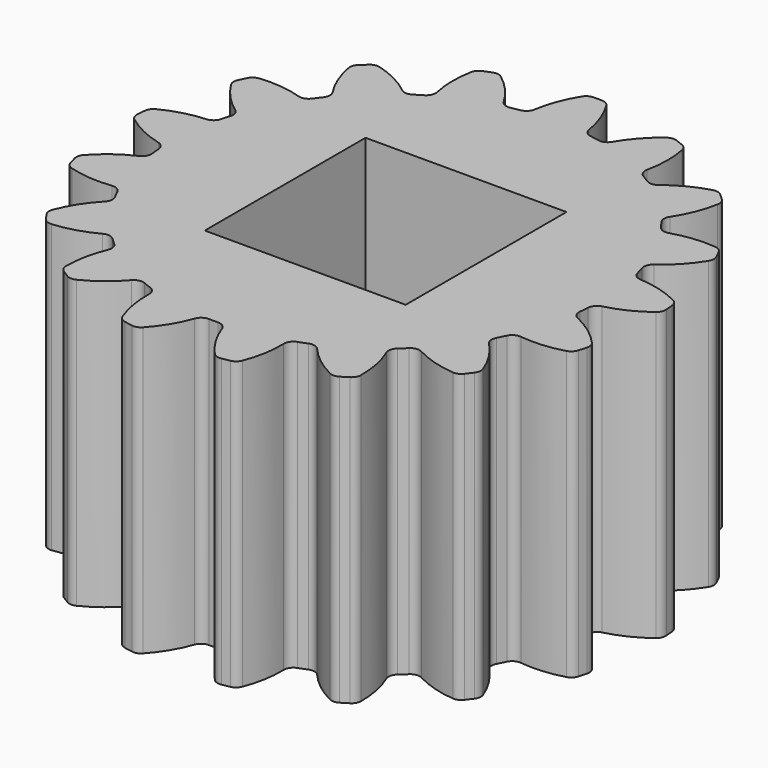
from build123d import *

# Parameters (mm, degrees)
F0_W            = 4.2
F0_H            = 4.2
F1_DEPTH        = 6
F2_DEPTH        = 6
F2_COPIES_COUNT = 16
F2_COPIES_ANGLE = 317.6470588235
F3_R            = 0.2


# Not quite as in the source:
# - a pattern or mirror of a feature is missing from the dataset's text; its kind, count and spacing are read off the source's solid


with BuildPart() as f1:
    # F0 (on Top) → F1 (new body)
    with BuildSketch(Plane.XY):
        with BuildLine():
            ThreePointArc((-0.587367865, 4.4615018762), (-2.967056168, -3.3832791337), (4.5, 0))
            ThreePointArc((4.5, 0), (3.3832791337, 2.967056168), (0.587367865, 4.4615018762))
            ThreePointArc((0.587367865, 4.4615018762), (0, 4.5), (-0.587367865, 4.4615018762))
        make_face()
        Rectangle(F0_W, F0_H, mode=Mode.SUBTRACT)
    extrude(amount=F1_DEPTH)

    # F0 (on Top) → F2 (join)
    with BuildSketch(Plane.XY):
        with BuildLine():
            ThreePointArc((-0.587367865, 4.4615018762), (0, 4.5), (0.587367865, 4.4615018762))
            ThreePointArc((0.587367865, 4.4615018762), (0.4600804215, 5.027237657), (0.1921950315, 5.5415298743))
            Line((0.1921950315, 5.5415298743), (-0.1921950315, 5.5415298743))
            ThreePointArc((-0.1921950315, 5.5415298743), (-0.4600804215, 5.027237657), (-0.587367865, 4.4615018762))
        make_face()
    f2 = extrude(amount=F2_DEPTH)

    # F2_copies: F2 ×16 about axis
    f2_copies_axis = Axis((0, 0, 0), (0, 0, -1))
    for i in range(1, F2_COPIES_COUNT):
        add(f2.rotate(f2_copies_axis, i * F2_COPIES_ANGLE / (F2_COPIES_COUNT - 1)))

    # F2_copies1: F2 across plane
    add(f2.mirror(Plane(origin=(0, 0, 0), x_dir=(0.1837494981, -0.9829731034, 0), z_dir=(-0.9829731034, -0.1837494981, 0))))

    # F3
    f3_edges = [f1.edges().sort_by_distance(p)[0] for p in [
        (-0.192195, 5.54153, 3),
        (-0.587368, 4.461502, 3),
        (0.192195, 5.54153, 3),
        (0.587368, 4.461502, 3),
        (4.451928, -0.656002, 3),
        (4.496665, -0.173207, 3),
        (5.382582, -1.331654, 3),
        (5.535624, 0.319933, 3),
        (5.500157, 0.702683, 3),
        (4.388274, 0.996518, 3),
        (4.255585, 1.462872, 3),
        (5.046243, 2.298026, 3),
        (4.874905, 2.642118, 3),
        (3.73196, 2.514453, 3),
        (3.439764, 2.901382, 3),
        (3.875338, 3.965759, 3),
        (3.591271, 4.224721, 3),
        (2.571624, 3.692797, 3),
        (2.159385, 3.948045, 3),
        (2.181048, 5.097894, 3),
        (1.822615, 5.236752, 3),
        (1.063976, 4.372408, 3),
        (-2.159384, 3.948045, 3),
        (-2.571624, 3.692797, 3),
        (-1.063976, 4.372408, 3),
        (-3.591271, 4.224721, 3),
        (-3.875338, 3.965759, 3),
        (-3.439764, 2.901382, 3),
        (-3.73196, 2.514453, 3),
        (-4.874905, 2.642118, 3),
        (-5.046243, 2.298026, 3),
        (-4.255585, 1.462872, 3),
        (-4.388274, 0.996518, 3),
        (-5.500157, 0.702683, 3),
        (-5.535624, 0.319933, 3),
        (-4.496665, -0.173207, 3),
        (-4.451928, -0.656002, 3),
        (-5.382582, -1.331654, 3),
        (-5.277389, -1.70137, 3),
        (-4.130446, -1.785893, 3),
        (-3.914324, -2.219926, 3),
        (-4.53806, -3.186143, 3),
        (-4.306413, -3.492893, 3),
        (-3.206387, -3.157385, 3),
        (-2.848068, -3.484036, 3),
        (-3.080647, -4.610326, 3),
        (-2.753832, -4.812681, 3),
        (-1.849288, -4.102455, 3),
        (-1.397166, -4.277608, 3),
        (-1.207176, -5.411859, 3),
        (-0.829331, -5.482491, 3),
        (-0.242432, -4.493465, 3),
        (0.242432, -4.493465, 3),
        (0.829331, -5.482491, 3),
        (1.207176, -5.411859, 3),
        (1.397166, -4.277608, 3),
        (1.849288, -4.102455, 3),
        (2.753832, -4.812681, 3),
        (3.080647, -4.610326, 3),
        (2.848068, -3.484036, 3),
        (3.206387, -3.157385, 3),
        (4.306413, -3.492893, 3),
        (4.53806, -3.186143, 3),
        (3.914324, -2.219926, 3),
        (4.130446, -1.785893, 3),
        (5.277389, -1.70137, 3),
        (-2.181048, 5.097894, 3),
        (-1.822615, 5.236752, 3),
    ]]
    fillet(f3_edges, radius=F3_R)


solid = f1.part
